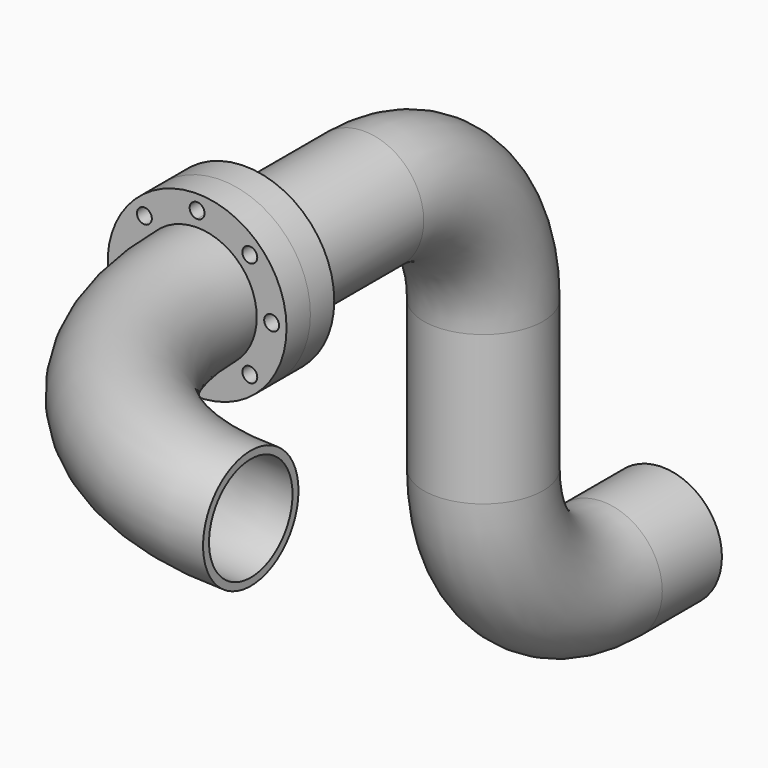
from build123d import *

# Parameters (mm, degrees)
F0_R     = 60
F0_R_2   = 5
F1_DEPTH = 20
F2_R     = 40
F2_R_2   = 35
F5_DEPTH = 20
F6_R     = 40
F6_R_2   = 35
F7_ANGLE = 90


with BuildPart() as f1:
    # F0 (on Front) → F1 (new body)
    with BuildSketch(Plane.XZ):
        Circle(F0_R)
        with Locations((-35.355339, -35.355339)):
            Circle(F0_R_2, mode=Mode.SUBTRACT)
        with Locations((0, -50)):
            Circle(F0_R_2, mode=Mode.SUBTRACT)
        with Locations((35.355339, -35.355339)):
            Circle(F0_R_2, mode=Mode.SUBTRACT)
        with Locations((-50, 0)):
            Circle(F0_R_2, mode=Mode.SUBTRACT)
        with Locations((-35.355339, 35.355339)):
            Circle(F0_R_2, mode=Mode.SUBTRACT)
        with BuildLine():
            ThreePointArc((35, 0), (-24.748737, -24.748737), (0, 35))
            ThreePointArc((0, 35), (24.748737, 24.748737), (35, 0))
        make_face(mode=Mode.SUBTRACT)
        with Locations((50, 0)):
            Circle(F0_R_2, mode=Mode.SUBTRACT)
        with BuildLine():
            ThreePointArc((0, 45), (-3.535534, 53.535534), (5, 50))
            ThreePointArc((5, 50), (3.535534, 46.464466), (0, 45))
        make_face(mode=Mode.SUBTRACT)
        with Locations((35.355339, 35.355339)):
            Circle(F0_R_2, mode=Mode.SUBTRACT)
    extrude(amount=F1_DEPTH)

    # F4: sweep along a path in F3
    with BuildLine(Plane.YZ) as f4_path:
        Line((0, 0), (100, 0))
        ThreePointArc((100, 0), (170.710678, -29.289322), (200, -100))
        Line((200, -100), (200, -200))
        ThreePointArc((200, -200), (229.289322, -270.710678), (300, -300))
        Line((300, -300), (350, -300))
    # F2 (on Front) → F4 (sweep)
    with BuildSketch(Plane.XZ):
        Circle(F2_R)
        Circle(F2_R_2, mode=Mode.SUBTRACT)
    sweep(path=f4_path.line)


with BuildPart() as f5:
    # F5 (new): a face of the model
    f5_faces = [f1.part.faces().sort_by_distance(p)[0] for p in [
        (-58.302944, -20, 0),
    ]]
    extrude(f5_faces, amount=F5_DEPTH)

    # F6 (on face) → F7 (revolve)
    with BuildSketch(Plane.XZ.offset(40)):
        Circle(F6_R)
        Circle(F6_R_2, mode=Mode.SUBTRACT)
    revolve(axis=Axis((180, -40, -12.128275), (0, 0, 1)), revolution_arc=F7_ANGLE)


solid = Compound([f1.part, f5.part])
